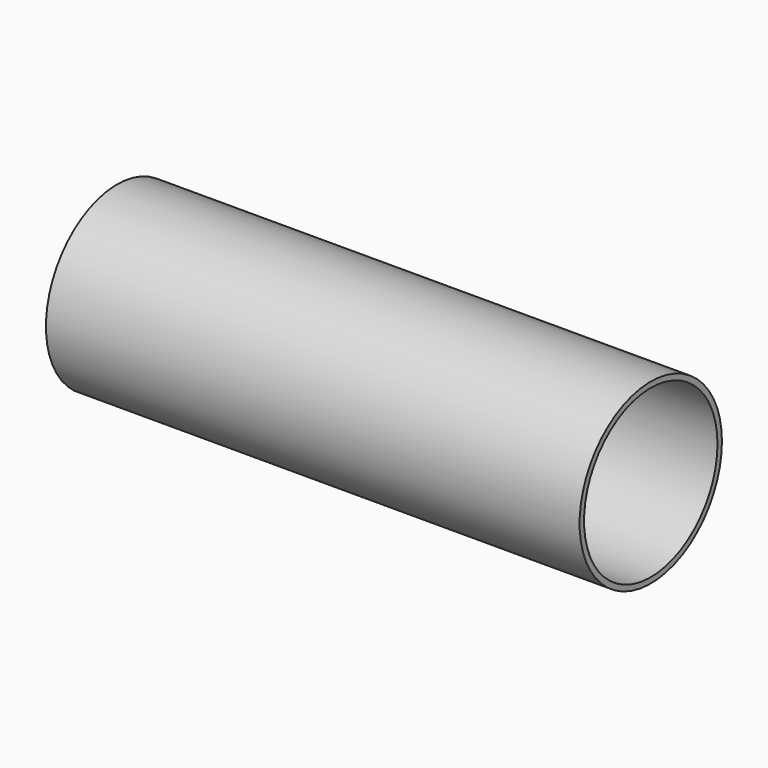
from build123d import *

# Parameters (mm, degrees)
F1_R     = 50.8
F1_R_2   = 47.625
F2_DEPTH = 304.8


# Not quite as in the source:
# - a variable given as a bare number and used for a length is read in inches; the dataset says mm whatever the document's units were


with BuildPart() as f2:
    # F1 (on Right) → F2 (new body)
    with BuildSketch(Plane.YZ):
        with Locations((13.9308627695, 20.094960928)):
            Circle(F1_R)
        with Locations((13.9308627695, 20.094960928)):
            Circle(F1_R_2, mode=Mode.SUBTRACT)
    extrude(amount=F2_DEPTH)


solid = f2.part
